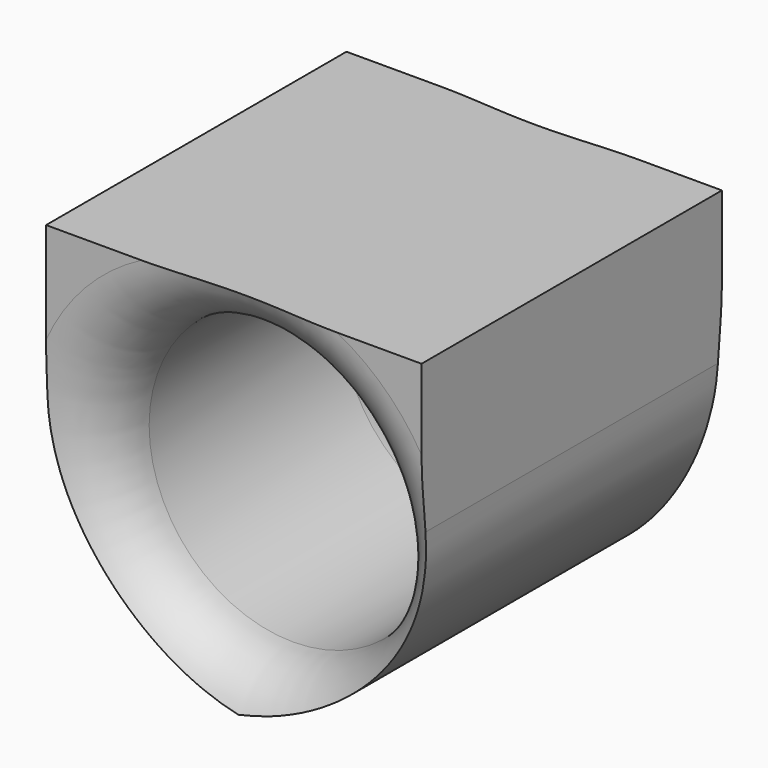
from build123d import *

# Parameters (mm, degrees)
F0_W        = 12.7
F0_H        = 12.7
F0_R        = 4.8737037562
F1_DEPTH    = 12.7
F3_T1_DEPTH = 50.8


# Not quite as in the source:
# - a fillet or chamfer that OpenCascade refuses, or shapes differently, is made with other operations: its cross-section is extruded or revolved along the edge and cut away or added


with BuildPart() as f1:
    # F0 (on Front) → F1 (new body)
    with BuildSketch(Plane.XZ):
        with Locations((-0.180745963, 2.9901557426)):
            Rectangle(F0_W, F0_H)
        with Locations((0, 2.9901557426)):
            Circle(F0_R, mode=Mode.SUBTRACT)
    extrude(amount=F1_DEPTH)

    # F2: fillet of radius 2.286 on 2 edges, made by hand

    # F2_s1 → F2_t2 (revolve, cut)
    with BuildSketch(Plane.XY.offset(2.9901557426)):
        with BuildLine():
            ThreePointArc((4.8737037562, -10.414), (5.5432576544, -12.0304461018), (7.1597037562, -12.7))
            Line((7.1597037562, -12.7), (4.8737037562, -12.7))
            Line((4.8737037562, -12.7), (4.8737037562, -10.414))
        make_face()
    revolve(axis=Axis((0, -12.7, 2.9901557426), (0, -1, 0)), mode=Mode.SUBTRACT)

    # F2_s3 → F2_t4 (revolve, cut)
    with BuildSketch(Plane.XY.offset(2.9901557426)):
        with BuildLine():
            ThreePointArc((4.8737037562, -2.286), (5.5432576544, -0.6695538982), (7.1597037562, 0))
            Line((7.1597037562, 0), (4.8737037562, 0))
            Line((4.8737037562, 0), (4.8737037562, -2.286))
        make_face()
    revolve(axis=Axis((0, 0, 2.9901557426), (0, -1, 0)), mode=Mode.SUBTRACT)

    # F3: fillet of radius 7.62 on 2 edges, made by hand

    # F3_s2 → F3_t1 (cut)
    with BuildSketch(Plane.XZ.offset(-19.05)):
        with BuildLine():
            ThreePointArc((6.169254037, 4.2601557426), (3.9374077096, -1.12799793), (-1.450745963, -3.3598442574))
            Line((-1.450745963, -3.3598442574), (6.169254037, -3.3598442574))
            Line((6.169254037, -3.3598442574), (6.169254037, 4.2601557426))
        make_face()
        with BuildLine():
            ThreePointArc((-6.530745963, 4.2601557426), (-4.2988996356, -1.12799793), (1.089254037, -3.3598442574))
            Line((1.089254037, -3.3598442574), (-6.530745963, -3.3598442574))
            Line((-6.530745963, -3.3598442574), (-6.530745963, 4.2601557426))
        make_face()
    extrude(amount=F3_T1_DEPTH, mode=Mode.SUBTRACT)


solid = f1.part
